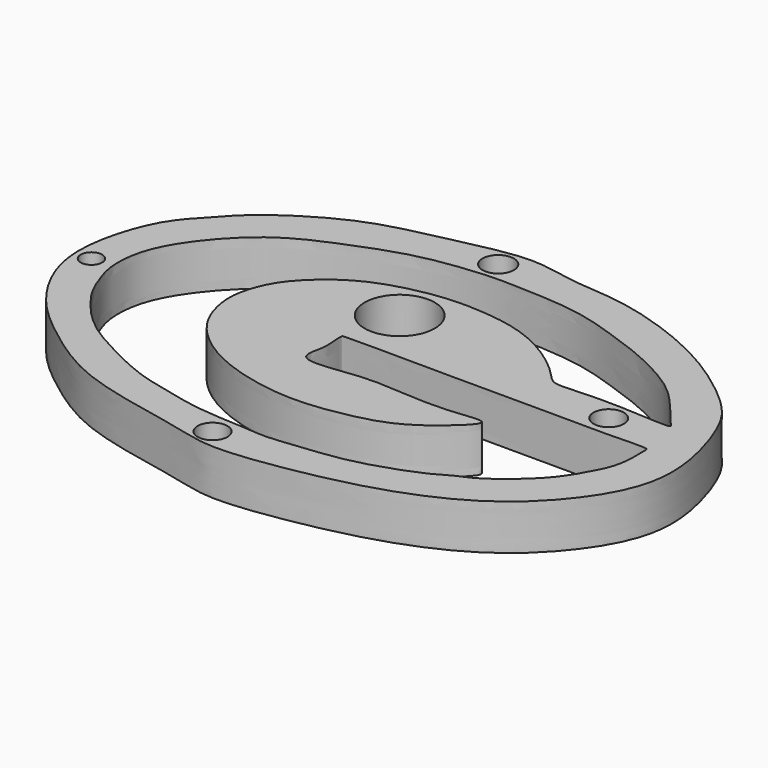
from build123d import *

# Parameters (mm, degrees)
F0_R     = 3.2852708183
F0_R_2   = 2.364425843
F0_R_3   = 7.7434653542
F0_R_4   = 3.4629833381
F0_R_5   = 3.3595828353
F1_DEPTH = 10


# Not quite as in the source:
# - a feature of the source that left no trace in its solid (it failed there, or was rolled back) is left out


with BuildPart() as f1:
    # F0 (on Top) → F1 (new body)
    with BuildSketch(Plane.XY):
        with BuildLine():
            add(Edge.make_bspline(
                [(64.0494674444, 17.5911355764), (62.7984905164, 20.4701002661), (59.9370782908, 25.0656361584), (48.589435907, 33.9650456559), (36.8879598008, 40.0849314506), (21.5840340204, 44.8993429065), (9.8520147184, 44.9047739559), (-0.0949793233, 47.9577091553), (-16.0255911483, 44.0687178402), (-30.2204308644, 41.2047061879), (-41.0991424388, 35.454020517), (-48.9659345942, 29.8302696852), (-54.1420970094, 24.0191545336), (-59.1528855447, 18.6549133838), (-63.1130787289, 7.9971655396), (-64.037236576, -4.7764253857), (-56.4293924574, -18.0798085839), (-45.8154494455, -26.6193009574), (-32.5966644484, -35.8342146024), (-9.4954986561, -39.4842663585), (-0.3455206577, -42.6918432339), (19.9552197096, -39.6893789454), (37.6769860623, -35.1252873549), (54.9124138985, -26.2376707258), (67.5873246573, -9.8369102569), (68.802420253, 3.7964859956), (65.6558142199, 13.8943322681), (64.0494674444, 17.5911355764)],
                knots=[0, 0, 0, 0, 0.0316957982, 0.0719785495, 0.112307218, 0.1555226318, 0.1923984551, 0.226751522, 0.2702879199, 0.3122347529, 0.3500465305, 0.3836814439, 0.4135651374, 0.4426623577, 0.4787561884, 0.5173293908, 0.5588234324, 0.5985682687, 0.6425803364, 0.694161984, 0.7285070984, 0.7763331596, 0.8236953482, 0.8712726428, 0.9195276041, 0.9593002539, 1, 1, 1, 1], degree=3))
        make_face()
        with Locations((-3.1871828251, -37.3166128993)):
            Circle(F0_R, mode=Mode.SUBTRACT)
        with Locations((-59.7596988082, 0)):
            Circle(F0_R_2, mode=Mode.SUBTRACT)
        with BuildLine():
            add(Edge.make_bspline(
                [(-7.9480279237, -5.5560898036), (-8.8169567089, -4.609224768), (-7.6053400325, -1.0133415387), (-7.9450891617, 1.1563250896), (-8.0739866503, 4.4624059763), (-7.8109743237, 4.4616155054), (-4.3925574508, 4.5419370966), (2.6445795495, 4.5431203801), (10.899584396, 4.3656826057), (17.2730845223, 4.48323533), (27.3988228529, 4.4669931534), (40.9791112485, 4.374903492), (49.9038437274, 4.2323068818), (59.0406328228, 4.6570933183), (59.4266509205, 4.0692972567), (59.4129227784, 1.963596855), (59.4792861123, -3.2964325057), (56.8706250426, -8.6422951546), (53.4415153232, -14.1863022628), (48.4940356249, -18.8226591037), (43.2564493038, -22.8071548224), (39.2793868065, -24.2201312216), (36.2876659284, -26.3202324233), (28.4391225859, -29.4004096684), (19.8903030292, -31.7311381151), (11.4116960673, -32.4180187612), (5.0220925418, -33.2869622899), (0.0174012007, -32.6708397783), (-10.0783065905, -32.4159277895), (-16.9867585758, -30.7084944119), (-26.0261590415, -28.8147658306), (-34.779092642, -24.5869296663), (-43.6288559237, -19.7815380815), (-49.0795691566, -13.8503069064), (-52.2560889397, -9.4115197408), (-54.2322068447, -4.4248570784), (-55.5489808464, 0.0698873522), (-55.0637837545, 8.7377443038), (-48.3610395553, 18.8666968707), (-39.4873310174, 27.0960742803), (-28.2056290546, 31.7510451479), (-16.2889161706, 36.3920060195), (-3.7175567234, 37.624993795), (-0.0191530353, 37.7744026449), (6.4787294615, 37.5923672982), (18.3469311645, 37.0345561054), (28.2250509812, 33.6689363307), (37.0451745339, 30.5797598502), (45.5931568616, 26.0326589173), (50.7548377762, 21.6449725117), (56.3003631351, 14.4796579761), (58.0295868679, 12.8953749238), (47.3886039912, 13.8519411722), (36.7668098679, 13.7579180807), (31.1141806188, 13.1419033459), (28.9150607451, 16.1612189664), (22.5167117484, 21.5044208246), (14.3358665683, 25.3780143883), (5.7486238398, 26.681501261), (-3.423778338, 26.9317714708), (-14.5428023516, 24.434385028), (-21.8325974304, 20.7035848022), (-28.5157722559, 14.6773186626), (-31.2533740192, 9.1307917713), (-32.6841543789, 3.2252277505), (-30.7000557185, -5.0114245762), (-25.5104222848, -10.9958001088), (-18.8457480598, -15.2966790445), (-9.9856263795, -18.3229400344), (0.0269460845, -19.5986661729), (9.4141739855, -18.4967011432), (19.1089722446, -16.16008698), (25.8039519708, -11.5308886807), (33.5949504452, -4.3318863991), (23.7455744872, -6.1406241402), (13.6393579036, -5.7895250881), (4.1291596333, -4.8134947984), (-6.5498046068, -7.0797230325), (-7.9480279237, -5.5560898036)],
                knots=[0, 0, 0, 0, 0.0100917886, 0.0183689929, 0.0265964706, 0.0282403898, 0.0365409801, 0.0500052787, 0.0640414375, 0.076296881, 0.0918384299, 0.1098060524, 0.1254221382, 0.1393094095, 0.1424076506, 0.1490523423, 0.1602709291, 0.1722318493, 0.1846564624, 0.197477888, 0.2100007884, 0.2197806345, 0.2289629891, 0.2429872297, 0.2578443538, 0.272125749, 0.2842691535, 0.2953035486, 0.3106319003, 0.3239261865, 0.33854515, 0.3539104211, 0.3694524359, 0.383193109, 0.3945777931, 0.4056617369, 0.4161419127, 0.4301147385, 0.4470809105, 0.4640369797, 0.4809300247, 0.4988460477, 0.5158504349, 0.5251061814, 0.5372083263, 0.5541643971, 0.5700534505, 0.5850493101, 0.5999557134, 0.6132724624, 0.6278845974, 0.6324822074, 0.6468580525, 0.6639938811, 0.6747670505, 0.6835460933, 0.6975422341, 0.7123927776, 0.7266283546, 0.7414989201, 0.7578505975, 0.7719720635, 0.7863864588, 0.7984018614, 0.8102371136, 0.824176592, 0.837803695, 0.8514424675, 0.8663558093, 0.8818351398, 0.8969087487, 0.9120600058, 0.9268995018, 0.9395192859, 0.9515611184, 0.9677169309, 0.9837609545, 1, 1, 1, 1], degree=3))
        make_face(mode=Mode.SUBTRACT)
        with Locations((-5.0463755615, 16.5999159217)):
            Circle(F0_R_3, mode=Mode.SUBTRACT)
        with Locations((-3.7183815148, 42.0973859727)):
            Circle(F0_R_4, mode=Mode.SUBTRACT)
        with Locations((47.0109693706, 9.1631542891)):
            Circle(F0_R_5, mode=Mode.SUBTRACT)
    extrude(amount=F1_DEPTH)


solid = f1.part
